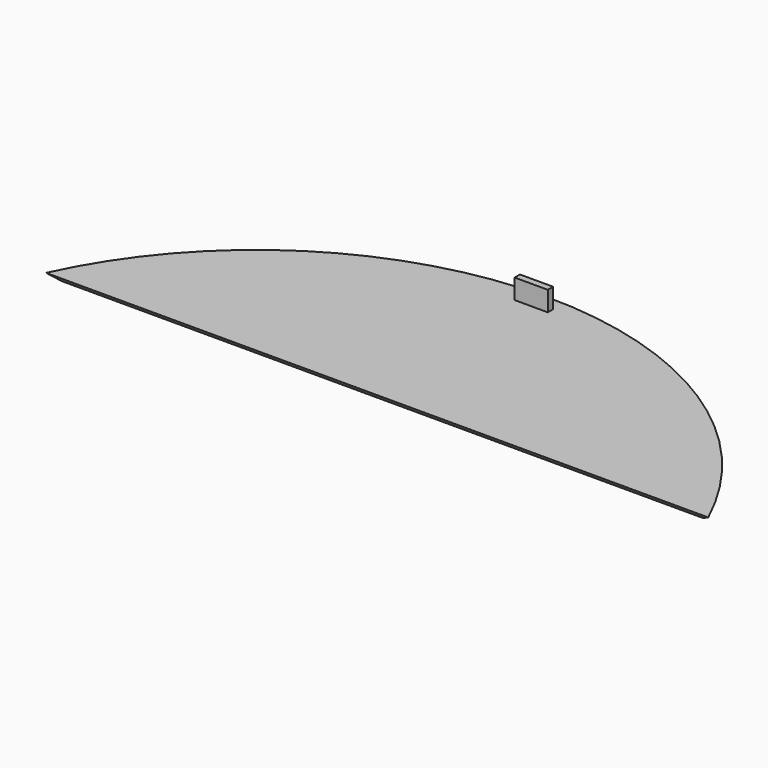
from build123d import *

# Parameters (mm, degrees)
F0_W     = 5
F0_H     = 1
F1_DEPTH = 4
F2_DEPTH = 1
F3_SIZE  = 0.99999


# Not quite as in the source:
# - a fillet or chamfer is up to 0.001 mm smaller than in the source, because OpenCascade refuses the exact size


with BuildPart() as f1:
    # F0 (on Top) → F1 (new body)
    with BuildSketch(Plane.XY):
        with Locations((0, 29.5871215252)):
            Rectangle(F0_W, F0_H)
    extrude(amount=F1_DEPTH)

    # F0 (on Top) → F2 (join)
    with BuildSketch(Plane.XY):
        with BuildLine():
            Line((-50, 0), (50, 0))
            ThreePointArc((50, 0), (0, 32.0871215252), (-50, 0))
        make_face()
        with Locations((0, 29.5871215252)):
            Rectangle(F0_W, F0_H, mode=Mode.SUBTRACT)
    extrude(amount=F2_DEPTH)

    # F3 (size 1 in the source; OpenCascade refuses exactly that, so slightly less here)
    f3_edges = [f1.edges().sort_by_distance(p)[0] for p in [
        (0, 32.087122, 0),
        (0, 0, 0),
    ]]
    chamfer(f3_edges, length=F3_SIZE)


solid = f1.part
